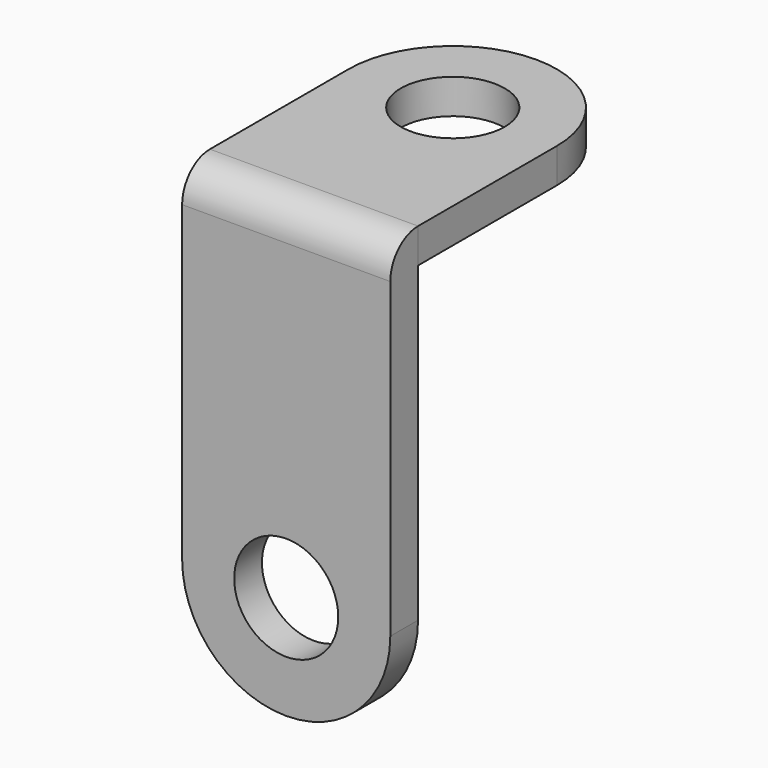
from build123d import *

# Parameters (mm, degrees)
F0_R     = 1.5
F1_DEPTH = 1
F2_R     = 1.5
F3_DEPTH = 1
F4_R     = 0.99999


# Not quite as in the source:
# - a fillet or chamfer is up to 0.001 mm smaller than in the source, because OpenCascade refuses the exact size


with BuildPart() as f1:
    # F0 (on Front) → F1 (new body)
    with BuildSketch(Plane.XZ):
        with BuildLine():
            Line((-0.3448204223, 13), (-0.3448204223, 3))
            ThreePointArc((-0.3448204223, 3), (0.5338592341, 0.8786796564), (2.6551795777, 0))
            ThreePointArc((2.6551795777, 0), (4.7764999212, 0.8786796564), (5.6551795777, 3))
            Line((5.6551795777, 3), (5.6551795777, 13))
            Line((5.6551795777, 13), (-0.3448204223, 13))
        make_face()
        with Locations((2.6551795777, 3)):
            Circle(F0_R, mode=Mode.SUBTRACT)
    extrude(amount=F1_DEPTH)

    # F4 (radius 1 in the source; OpenCascade refuses exactly that, so slightly less here)
    f4_edges = [f1.edges().sort_by_distance(p)[0] for p in [
        (2.65518, -1, 13),
    ]]
    fillet(f4_edges, radius=F4_R)


with BuildPart() as f3:
    # F2 (on face) → F3 (new body)
    with BuildSketch(Plane.XY.offset(13)):
        with BuildLine():
            Line((-0.3448204223, 5), (-0.3448204223, 0))
            Line((-0.3448204223, 0), (5.6551795777, 0))
            Line((5.6551795777, 0), (5.6551795777, 5))
            ThreePointArc((5.6551795777, 5), (2.6551795777, 8), (-0.3448204223, 5))
        make_face()
        with Locations((2.6551795777, 5)):
            Circle(F2_R, mode=Mode.SUBTRACT)
    extrude(amount=-F3_DEPTH)


solid = Compound([f1.part, f3.part])
